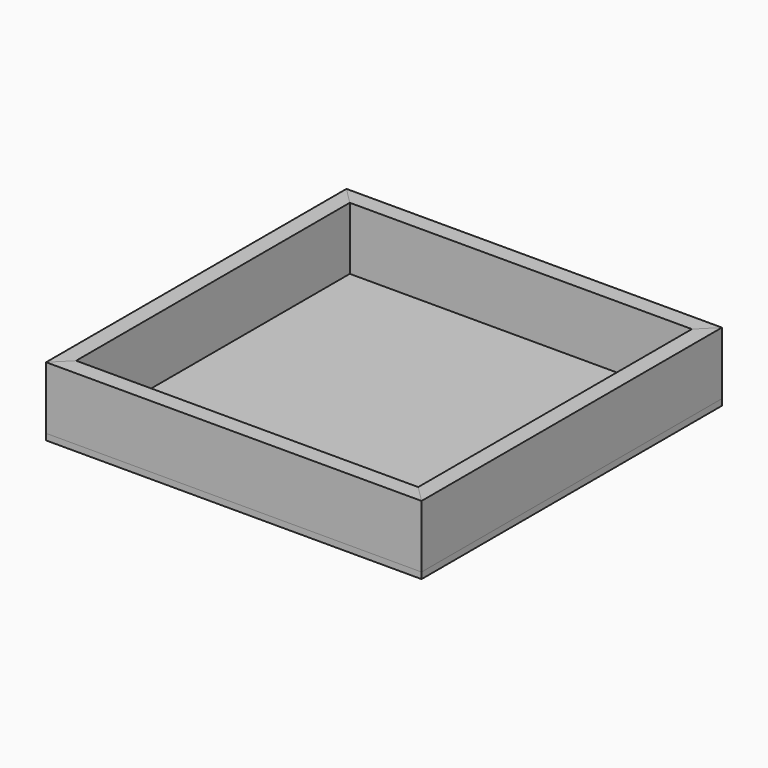
from build123d import *

# Parameters (mm, degrees)
F0_W     = 180
F0_H     = 180
F1_DEPTH = 3
F3_DEPTH = 30
F4_DEPTH = 30
F5_DEPTH = 30
F6_DEPTH = 30


# Not quite as in the source:
# - an extrude ends at something that could not be found from the text; its depth is read off the source's solid


with BuildPart() as f1:
    # F0 (on Top) → F1 (new body)
    with BuildSketch(Plane.XY):
        with Locations((90, 90)):
            Rectangle(F0_W, F0_H)
    extrude(amount=F1_DEPTH)


with BuildPart() as f3:
    # F2 (on face) → F3 (new body)
    with BuildSketch(Plane.XY.offset(3)):
        Polygon((0, 180), (8, 172), (172, 172), (180, 180), align=None)
    extrude(amount=F3_DEPTH)


with BuildPart() as f4:
    # F2 (on face) → F4 (new body, through all)
    with BuildSketch(Plane.XY.offset(3)):
        Polygon((180, 180), (172, 172), (172, 8), (180, 0), align=None)
    extrude(amount=F4_DEPTH)


with BuildPart() as f5:
    # F2 (on face) → F5 (new body, through all)
    with BuildSketch(Plane.XY.offset(3)):
        Polygon((172, 8), (8, 8), (0, 0), (180, 0), align=None)
    extrude(amount=F5_DEPTH)


with BuildPart() as f6:
    # F2 (on face) → F6 (new body, through all)
    with BuildSketch(Plane.XY.offset(3)):
        Polygon((8, 8), (8, 172), (0, 180), (0, 0), align=None)
    extrude(amount=F6_DEPTH)


solid = Compound([f1.part, f3.part, f4.part, f5.part, f6.part])
